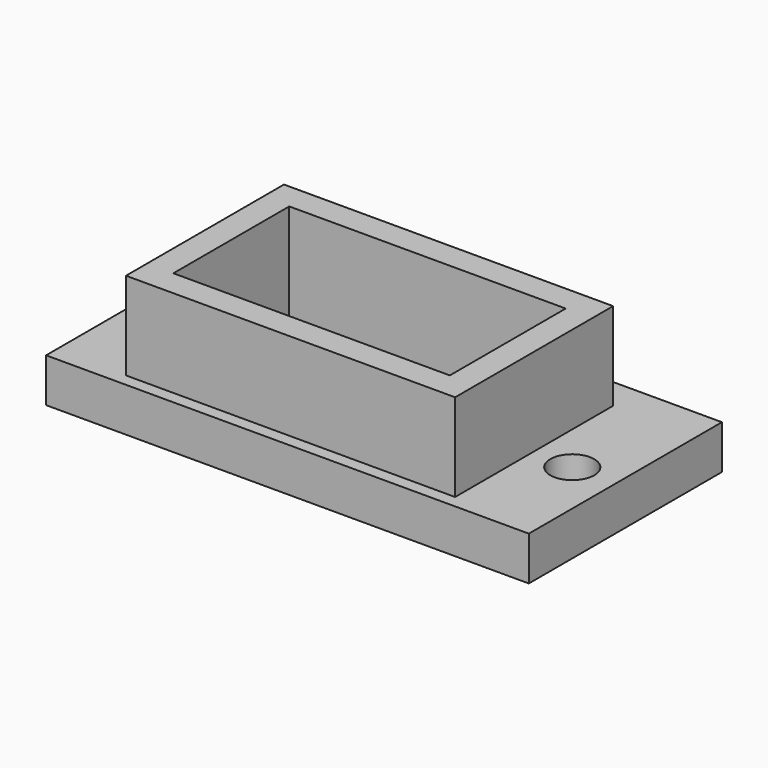
from build123d import *

# Parameters (mm, degrees)
F0_W        = 22
F0_H        = 11
F1_DEPTH    = 2
F2_W        = 15
F2_H        = 9
F3_DEPTH    = 6
F4_T        = 1.2
F4_T3_DEPTH = 17.4
F4_T5_DEPTH = 11.4
F6_R        = 1
F7_DEPTH    = 25
F5_R        = 1
F8_DEPTH    = 25


# Not quite as in the source:
# - a shell that OpenCascade refuses in one call is made with other operations: the cavity is built on its own and cut out


with BuildPart() as f1:
    # F0 (on Top) → F1 (new body)
    with BuildSketch(Plane.XY):
        with Locations((10.5796571493, 0.5358164497)):
            Rectangle(F0_W, F0_H)
    extrude(amount=F1_DEPTH)

    # F2 (on Top) → F3 (join)
    with BuildSketch(Plane.XY):
        with Locations((10.2674138546, 0.1021951512)):
            Rectangle(F2_W, F2_H)
    extrude(amount=F3_DEPTH)

    # F4: shell of thickness 1.2, made by hand


with BuildPart() as f4_core1:
    # F4_t2: copy of F1
    add(f1.part)

    # the walls: a layer under each face that stays
    f4_faces = [f4_core1.faces().sort_by_distance(p)[0] for p in [
        (10.5796571493, -4.9641835503, 1),
        (-0.4203428507, 0.5358164497, 1),
        (21.5796571493, 0.5358164497, 1),
        (10.5796571493, 0.5358164497, 0),
        (17.9129904826, -3.130850217, 2),
        (10.5796571493, 6.0358164497, 1),
        (10.2674138546, -4.3978048488, 4),
        (17.7674138546, 0.1021951512, 4),
        (10.2674138546, 4.6021951512, 4),
        (2.7674138546, 0.1021951512, 4),
    ]]
    thicken(f4_faces, amount=-F4_T, mode=Mode.SUBTRACT)

    # F4_s4 → F4_t3 (cut)
    with BuildSketch(Plane.YZ.offset(1.5674138546)):
        Polygon((-4.4098048488, 2.012), (-4.3978048488, 0.8), (-3.1978048488, 0.8), (-3.1978048488, 2), align=None)
        Polygon((4.6141951512, 2.012), (4.6021951512, 0.8), (3.4021951512, 0.8), (3.4021951512, 2), align=None)
    extrude(amount=F4_T3_DEPTH, mode=Mode.SUBTRACT)

    # F4_s6 → F4_t5 (cut)
    with BuildSketch(Plane.XZ.offset(-5.8021951512)):
        Polygon((17.7794138546, 2.012), (17.7674138546, 0.8), (16.5674138546, 0.8), (16.5674138546, 2), align=None)
        Polygon((2.7554138546, 2.012), (2.7674138546, 0.8), (3.9674138546, 0.8), (3.9674138546, 2), align=None)
    extrude(amount=F4_T5_DEPTH, mode=Mode.SUBTRACT)


with BuildPart() as f1_1:
    add(f1.part)

    # what is left inside the walls is the cavity
    f4_cavity = [f4_core1.part.solids().sort_by_distance(p)[0] for p in [
        (10.267414, -0.997805, 1.212),
    ]]
    add(f4_cavity, mode=Mode.SUBTRACT)

    # F6 (on face) → F7 (cut)
    with BuildSketch(Plane.XY.offset(2)):
        with Locations((19.5883829147, 0)):
            Circle(F6_R)
    extrude(amount=-F7_DEPTH, mode=Mode.SUBTRACT)

    # F5 (on face) → F8 (cut)
    with BuildSketch(Plane.XY.offset(2)):
        with Locations((1.0301771374, -0.018063417)):
            Circle(F5_R)
    extrude(amount=-F8_DEPTH, mode=Mode.SUBTRACT)


solid = f1_1.part
